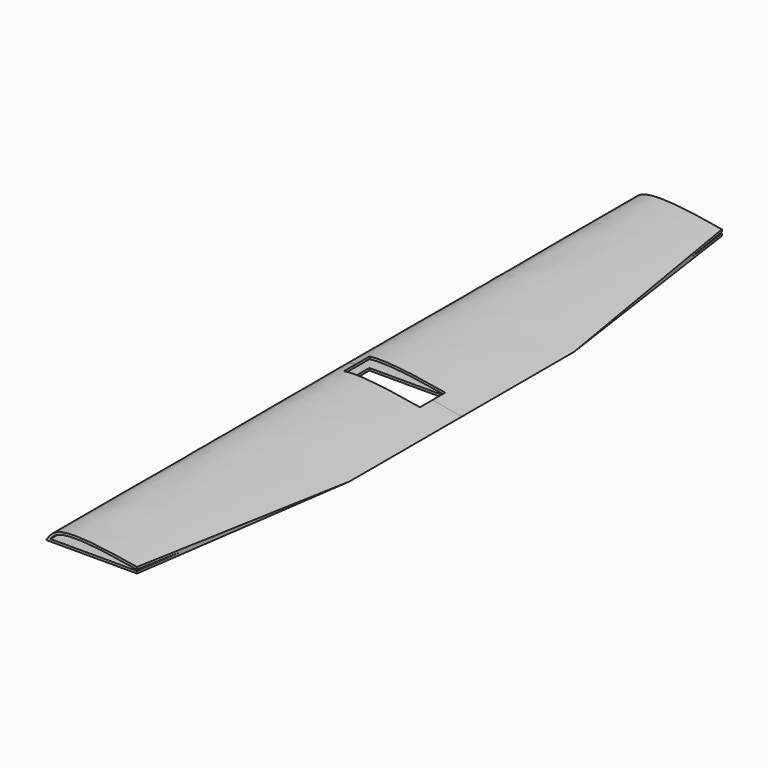
from build123d import *

# Parameters (mm, degrees)
F2_DEPTH = 173.3
F4_DEPTH = 25
F6_W     = 36
F6_H     = 15
F7_DEPTH = 20


# Not quite as in the source:
# - ends of sketch curves that miss each other by under 0.0002 mm in the source are joined
# - the dataset's text gives a spline's control points without its knots; the knots are read off the source's solid


with BuildPart() as f2:
    # F1 (on face) → F2 (new body)
    with BuildSketch(Plane.XZ):
        with BuildLine():
            add(Edge.make_bspline(
                [(-26.5921223909, 0), (-25.2176326426, 2.1217019965), (-20.3510980326, 9.6338251033), (10.0223686099, 4.0248166048), (31.8172425032, 0)],
                knots=[0, 0, 0, 0, 0.2824370642, 1, 1, 1, 1], degree=3))
            Line((-26.5921223909, 0), (31.8172425032, 0))
        make_face()
        with BuildLine():
            add(Edge.make_bspline(
                [(19.6565909304, 1.0999999067), (16.1575857425, 1.7220457641), (9.0829705679, 2.9345711326), (0.8605637985, 4.1185996724), (-5.2320226887, 4.7661728451), (-9.4250497651, 5.0645366103), (-13.1839026492, 5.150174403), (-15.9032026434, 5.0246144265), (-17.7956903302, 4.7976821367), (-19.064531223, 4.5634552716), (-20.1691059627, 4.2672043663), (-21.4253720439, 3.7905449175), (-22.667375377, 3.0608525064), (-23.7126545919, 2.1017508626), (-24.2810764737, 1.407206711), (-24.5122916533, 1.0999768794)],
                knots=[0.1322462263, 0.1322462263, 0.1322462263, 0.1322462263, 0.25, 0.375, 0.4375, 0.5, 0.5625, 0.625, 0.65625, 0.6875, 0.71875, 0.75, 0.8125, 0.875, 0.9208192438, 0.9208192438, 0.9208192438, 0.9208192438], degree=3))
            Line((19.6565909304, 1.0999999067), (-24.5122916533, 1.0999768794))
        make_face(mode=Mode.SUBTRACT)
    extrude(amount=F2_DEPTH)

    # F3 (on Top) → F4 (cut)
    with BuildSketch(Plane.XY):
        Polygon((65.3333365917, -177.500128746), (42.7832975984, 10.0049925968), (15.9085858613, -177.500128746), align=None)
    extrude(amount=F4_DEPTH, mode=Mode.SUBTRACT)

    # F5: F2 across plane


with BuildPart() as f2_1:
    add(f2.part)
    add(f2.part.mirror(Plane.XZ))

    # F6 (on Top) → F7 (cut)
    with BuildSketch(Plane.XY):
        Rectangle(F6_W, F6_H)
    extrude(amount=F7_DEPTH, mode=Mode.SUBTRACT)


solid = f2_1.part
